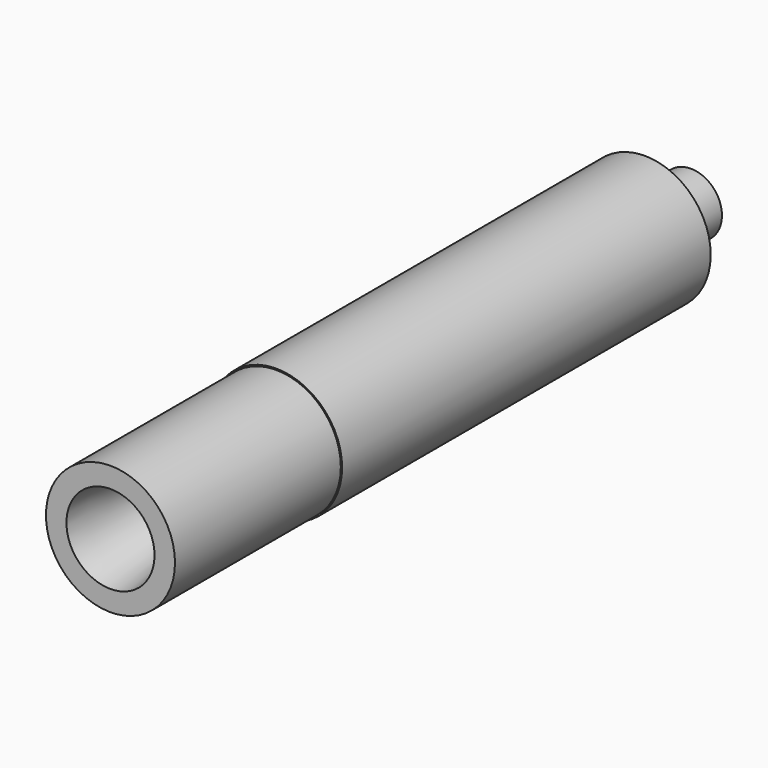
from build123d import *

# Parameters (mm, degrees)
F0_R      = 12.7
F0_R_2    = 6.35
F1_DEPTH  = 88.9
F2_R      = 12.45
F3_DEPTH  = 40
F4_R      = 8.5
F5_DEPTH  = 30
F5_TAPER  = 8
F6_R      = 6
F7_DEPTH  = 100
F8_R      = 3.96875
F9_DEPTH  = 140.0010001
F10_R     = 10.5
F11_DEPTH = 5
F12_R     = 10.5
F12_R_2   = 6
F13_DEPTH = 5
F14_R     = 10.5
F15_DEPTH = 5
F16_R     = 10.5
F16_R_2   = 6
F17_DEPTH = 5


with BuildPart() as f1:
    # F0 (on Front) → F1 (new body)
    with BuildSketch(Plane.XZ):
        Circle(F0_R)
        Circle(F0_R_2, mode=Mode.SUBTRACT)
    extrude(amount=-F1_DEPTH)

    # F10 (on face) → F11 (cut)
    with BuildSketch(Plane.XZ):
        Circle(F10_R)
    extrude(amount=-F11_DEPTH, mode=Mode.SUBTRACT)

    # F14 (on face) → F15 (cut)
    with BuildSketch(Plane(origin=(0, 88.9, 0), x_dir=(-1, 0, 0), z_dir=(0, 1, 0))):
        Circle(F14_R)
    extrude(amount=-F15_DEPTH, mode=Mode.SUBTRACT)


with BuildPart() as f3:
    # F2 (on Front) → F3 (new body)
    with BuildSketch(Plane.XZ):
        Circle(F2_R)
    extrude(amount=F3_DEPTH)

    # F4 (on face) → F5 (cut)
    with BuildSketch(Plane.XZ.offset(40)):
        Circle(F4_R)
    extrude(amount=-F5_DEPTH, taper=F5_TAPER, mode=Mode.SUBTRACT)

    # F6 (on face) → F7 (join)
    with BuildSketch(Plane(origin=(0, 0, 0), x_dir=(-1, 0, 0), z_dir=(0, 1, 0))):
        Circle(F6_R)
    extrude(amount=F7_DEPTH)

    # F8 (on face) → F9 (cut, through all)
    with BuildSketch(Plane(origin=(0, 100, 0), x_dir=(-1, 0, 0), z_dir=(0, 1, 0))):
        Circle(F8_R)
    extrude(amount=-F9_DEPTH, mode=Mode.SUBTRACT)


with BuildPart() as f13:
    # F12 (on face) → F13 (new body)
    with BuildSketch(Plane.XZ.offset(-5)):
        Circle(F12_R)
        Circle(F12_R_2, mode=Mode.SUBTRACT)
    extrude(amount=F13_DEPTH)


with BuildPart() as f17:
    # F16 (on face) → F17 (new body)
    with BuildSketch(Plane(origin=(0, 83.9, 0), x_dir=(-1, 0, 0), z_dir=(0, 1, 0))):
        Circle(F16_R)
        Circle(F16_R_2, mode=Mode.SUBTRACT)
    extrude(amount=F17_DEPTH)


solid = Compound([f1.part, f3.part, f13.part, f17.part])
